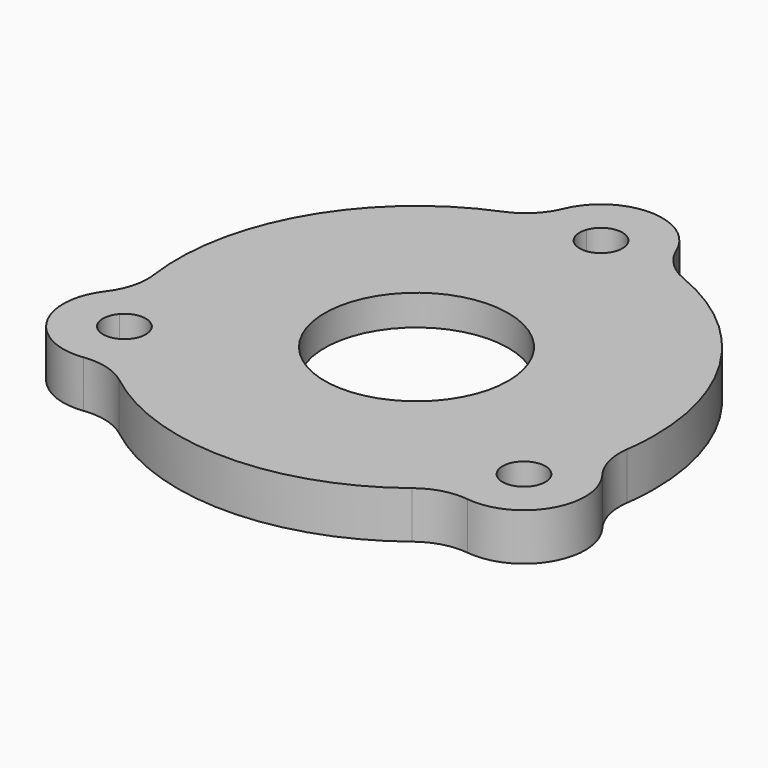
from build123d import *

# Parameters (mm, degrees)
F1_DEPTH = 1.7145
F0_R     = 9.525
F2_DEPTH = 3.175
F3_R     = 6.35
F4_R     = 5.08


with BuildPart() as f1:
    # F0 (on Top) → F1 (new body)
    with BuildSketch(Plane.XY):
        with BuildLine():
            ThreePointArc((23.9050999455, -6.4692674698), (24.5490837421, -3.2630832697), (24.765, 0))
            ThreePointArc((24.765, 0), (19.6285885254, 15.1004548773), (6.35, 23.9370575677))
            ThreePointArc((6.35, 23.9370575677), (4.2391432725, 24.3994854314), (2.0960107473, 24.6761415936))
            ThreePointArc((2.0960107473, 24.6761415936), (2.1906494626, 24.3119724675), (2.2225, 23.9370575677))
            ThreePointArc((2.2225, 23.9370575677), (-0.3749148998, 21.7464081051), (-2.0960107473, 24.6761415936))
            ThreePointArc((-2.0960107473, 24.6761415936), (-4.2391432725, 24.3994854314), (-6.35, 23.9370575677))
            ThreePointArc((-6.35, 23.9370575677), (-21.4471191247, 12.3825), (-23.9050999455, -6.4692674698))
            ThreePointArc((-23.9050999455, -6.4692674698), (-23.2501458591, -8.5285369514), (-22.4181708611, -10.5228722431))
            ThreePointArc((-22.4181708611, -10.5228722431), (-19.9594610417, -9.8839132486), (-18.5075999455, -11.9685287839))
            ThreePointArc((-18.5075999455, -11.9685287839), (-19.02039931, -13.3885393426), (-20.3221601138, -14.1532693505))
            ThreePointArc((-20.3221601138, -14.1532693505), (-19.0110025866, -15.87094848), (-17.5550999455, -17.4677900979))
            ThreePointArc((-17.5550999455, -17.4677900979), (0, -24.765), (17.5550999455, -17.4677900979))
            ThreePointArc((17.5550999455, -17.4677900979), (19.0110025866, -15.87094848), (20.3221601138, -14.1532693505))
            ThreePointArc((20.3221601138, -14.1532693505), (18.8053584856, -10.8572787839), (22.4181708611, -10.5228722431))
            ThreePointArc((22.4181708611, -10.5228722431), (23.2501458591, -8.5285369514), (23.9050999455, -6.4692674698))
        make_face()
        with BuildLine():
            ThreePointArc((-6.35, -11.7260276735), (-6.8244038201, 11.4564277809), (13.335, 0))
            ThreePointArc((13.335, 0), (11.4564277809, -6.8244038201), (6.35, -11.7260276735))
            Line((6.35, -11.7260276735), (6.35, -20.955))
            Line((6.35, -20.955), (-6.35, -20.955))
            Line((-6.35, -20.955), (-6.35, -11.7260276735))
        make_face(mode=Mode.SUBTRACT)
        with BuildLine():
            ThreePointArc((2.0960107473, 24.6761415936), (4.2391432725, 24.3994854314), (6.35, 23.9370575677))
            ThreePointArc((6.35, 23.9370575677), (0, 30.2870575677), (-6.35, 23.9370575677))
            ThreePointArc((-6.35, 23.9370575677), (-4.2391432725, 24.3994854314), (-2.0960107473, 24.6761415936))
            ThreePointArc((-2.0960107473, 24.6761415936), (0, 26.1595575677), (2.0960107473, 24.6761415936))
        make_face()
        with BuildLine():
            ThreePointArc((17.5550999455, -17.4677900979), (26.2293612595, -15.1435287839), (23.9050999455, -6.4692674698))
            ThreePointArc((23.9050999455, -6.4692674698), (23.2501458591, -8.5285369514), (22.4181708611, -10.5228722431))
            ThreePointArc((22.4181708611, -10.5228722431), (22.8147154808, -11.1978898801), (22.9525999455, -11.9685287839))
            ThreePointArc((22.9525999455, -11.9685287839), (22.1501105043, -13.6782294193), (20.3221601138, -14.1532693505))
            ThreePointArc((20.3221601138, -14.1532693505), (19.0110025866, -15.87094848), (17.5550999455, -17.4677900979))
        make_face()
        with BuildLine():
            ThreePointArc((-22.4181708611, -10.5228722431), (-23.2501458591, -8.5285369514), (-23.9050999455, -6.4692674698))
            ThreePointArc((-23.9050999455, -6.4692674698), (-26.2293612595, -15.1435287839), (-17.5550999455, -17.4677900979))
            ThreePointArc((-17.5550999455, -17.4677900979), (-19.0110025866, -15.87094848), (-20.3221601138, -14.1532693505))
            ThreePointArc((-20.3221601138, -14.1532693505), (-22.6548414054, -13.0797787839), (-22.4181708611, -10.5228722431))
        make_face()
    extrude(amount=-F1_DEPTH)

    # F0 (on Top) → F2 (join)
    with BuildSketch(Plane.XY):
        with BuildLine():
            ThreePointArc((23.9050999455, -6.4692674698), (24.5490837421, -3.2630832697), (24.765, 0))
            ThreePointArc((24.765, 0), (19.6285885254, 15.1004548773), (6.35, 23.9370575677))
            ThreePointArc((6.35, 23.9370575677), (4.2391432725, 24.3994854314), (2.0960107473, 24.6761415936))
            ThreePointArc((2.0960107473, 24.6761415936), (2.1906494626, 24.3119724675), (2.2225, 23.9370575677))
            ThreePointArc((2.2225, 23.9370575677), (-0.3749148998, 21.7464081051), (-2.0960107473, 24.6761415936))
            ThreePointArc((-2.0960107473, 24.6761415936), (-4.2391432725, 24.3994854314), (-6.35, 23.9370575677))
            ThreePointArc((-6.35, 23.9370575677), (-21.4471191247, 12.3825), (-23.9050999455, -6.4692674698))
            ThreePointArc((-23.9050999455, -6.4692674698), (-23.2501458591, -8.5285369514), (-22.4181708611, -10.5228722431))
            ThreePointArc((-22.4181708611, -10.5228722431), (-19.9594610417, -9.8839132486), (-18.5075999455, -11.9685287839))
            ThreePointArc((-18.5075999455, -11.9685287839), (-19.02039931, -13.3885393426), (-20.3221601138, -14.1532693505))
            ThreePointArc((-20.3221601138, -14.1532693505), (-19.0110025866, -15.87094848), (-17.5550999455, -17.4677900979))
            ThreePointArc((-17.5550999455, -17.4677900979), (0, -24.765), (17.5550999455, -17.4677900979))
            ThreePointArc((17.5550999455, -17.4677900979), (19.0110025866, -15.87094848), (20.3221601138, -14.1532693505))
            ThreePointArc((20.3221601138, -14.1532693505), (18.8053584856, -10.8572787839), (22.4181708611, -10.5228722431))
            ThreePointArc((22.4181708611, -10.5228722431), (23.2501458591, -8.5285369514), (23.9050999455, -6.4692674698))
        make_face()
        with BuildLine():
            ThreePointArc((-6.35, -11.7260276735), (-6.8244038201, 11.4564277809), (13.335, 0))
            ThreePointArc((13.335, 0), (11.4564277809, -6.8244038201), (6.35, -11.7260276735))
            Line((6.35, -11.7260276735), (6.35, -20.955))
            Line((6.35, -20.955), (-6.35, -20.955))
            Line((-6.35, -20.955), (-6.35, -11.7260276735))
        make_face(mode=Mode.SUBTRACT)
        with BuildLine():
            ThreePointArc((6.35, -11.7260276735), (11.4564277809, -6.8244038201), (13.335, 0))
            ThreePointArc((13.335, 0), (-6.8244038201, 11.4564277809), (-6.35, -11.7260276735))
            ThreePointArc((-6.35, -11.7260276735), (0, -13.335), (6.35, -11.7260276735))
        make_face()
        Circle(F0_R, mode=Mode.SUBTRACT)
        with BuildLine():
            ThreePointArc((6.35, -11.7260276735), (0, -13.335), (-6.35, -11.7260276735))
            Line((-6.35, -11.7260276735), (-6.35, -20.955))
            Line((-6.35, -20.955), (6.35, -20.955))
            Line((6.35, -20.955), (6.35, -11.7260276735))
        make_face()
        with BuildLine():
            ThreePointArc((2.0960107473, 24.6761415936), (4.2391432725, 24.3994854314), (6.35, 23.9370575677))
            ThreePointArc((6.35, 23.9370575677), (0, 30.2870575677), (-6.35, 23.9370575677))
            ThreePointArc((-6.35, 23.9370575677), (-4.2391432725, 24.3994854314), (-2.0960107473, 24.6761415936))
            ThreePointArc((-2.0960107473, 24.6761415936), (0, 26.1595575677), (2.0960107473, 24.6761415936))
        make_face()
        with BuildLine():
            ThreePointArc((-22.4181708611, -10.5228722431), (-23.2501458591, -8.5285369514), (-23.9050999455, -6.4692674698))
            ThreePointArc((-23.9050999455, -6.4692674698), (-26.2293612595, -15.1435287839), (-17.5550999455, -17.4677900979))
            ThreePointArc((-17.5550999455, -17.4677900979), (-19.0110025866, -15.87094848), (-20.3221601138, -14.1532693505))
            ThreePointArc((-20.3221601138, -14.1532693505), (-22.6548414054, -13.0797787839), (-22.4181708611, -10.5228722431))
        make_face()
        with BuildLine():
            ThreePointArc((17.5550999455, -17.4677900979), (26.2293612595, -15.1435287839), (23.9050999455, -6.4692674698))
            ThreePointArc((23.9050999455, -6.4692674698), (23.2501458591, -8.5285369514), (22.4181708611, -10.5228722431))
            ThreePointArc((22.4181708611, -10.5228722431), (22.8147154808, -11.1978898801), (22.9525999455, -11.9685287839))
            ThreePointArc((22.9525999455, -11.9685287839), (22.1501105043, -13.6782294193), (20.3221601138, -14.1532693505))
            ThreePointArc((20.3221601138, -14.1532693505), (19.0110025866, -15.87094848), (17.5550999455, -17.4677900979))
        make_face()
    extrude(amount=F2_DEPTH)

    # F3
    f3_edges = [f1.edges().sort_by_distance(p)[0] for p in [
        (-23.9051, -6.469267, -0.85725),
        (6.35, 23.937058, 0.73025),
        (17.5551, -17.46779, 0.73025),
        (23.9051, -6.469267, 0.73025),
        (-17.5551, -17.46779, -0.85725),
        (-17.5551, -17.46779, 1.5875),
        (-23.9051, -6.469267, 1.5875),
        (-6.35, 23.937058, 1.5875),
        (-6.35, 23.937058, -0.85725),
    ]]
    fillet(f3_edges, radius=F3_R)

    # F4
    f4_edges = [f1.edges().sort_by_distance(p)[0] for p in [
        (-6.35, -11.726028, -0.85725),
        (6.35, -11.726028, -0.85725),
        (6.35, -20.955, -0.85725),
        (-6.35, -20.955, -0.85725),
    ]]
    fillet(f4_edges, radius=F4_R)


solid = f1.part
